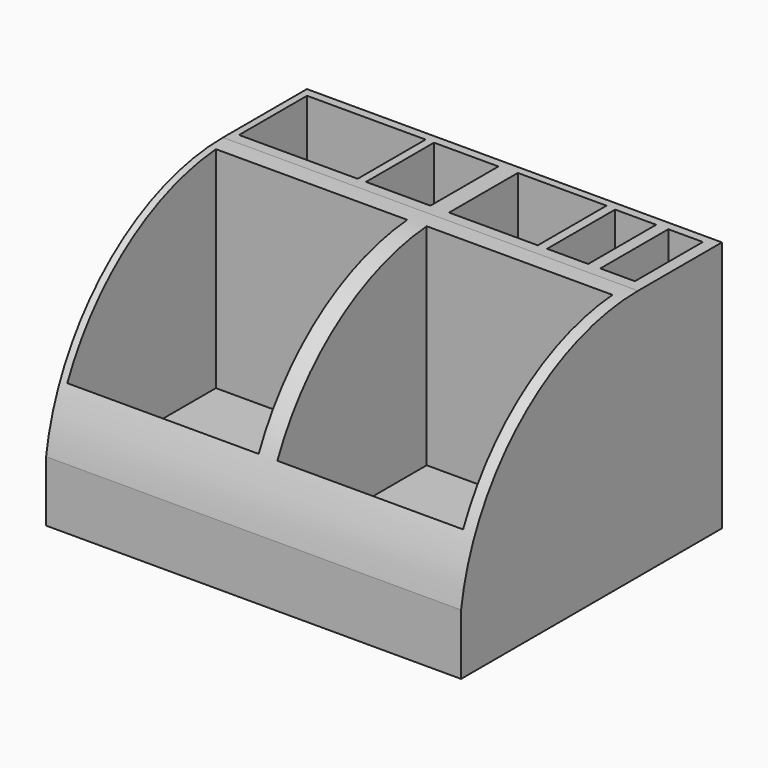
from build123d import *

# Parameters (mm, degrees)
F0_W        = 142.3350870609
F0_H        = 111.8143312633
F1_DEPTH    = 65.532
F2_T1_DEPTH = 521.5375533391
F4_DEPTH    = 20.828
F3_W        = 65.6352208462
F3_H        = 63.7141903862
F3_W_2      = 63.7141834013
F3_H_2      = 64.0343613923
F3_W_3      = 30.4163205437
F3_H_3      = 29.4558089226
F3_W_4      = 22.0918541308
F3_H_4      = 29.1356351227
F3_W_5      = 14.0875652432
F3_W_6      = 11.8463523686
F3_W_7      = 40.6618192792
F5_DEPTH    = 72.39


# Not quite as in the source:
# - a fillet or chamfer that OpenCascade refuses, or shapes differently, is made with other operations: its cross-section is extruded or revolved along the edge and cut away or added


with BuildPart() as f1:
    # F0 (on Top) → F1 (new body)
    with BuildSketch(Plane.XY):
        with Locations((-0.4278570414, 0.1426208764)):
            Rectangle(F0_W, F0_H)
    extrude(amount=F1_DEPTH)

    # F2: fillet of radius 76.6512806053 on 1 edges, made by hand

    # F2_s2 → F2_t1 (cut)
    with BuildSketch(Plane.YZ.offset(-261.1966337109)):
        with BuildLine():
            ThreePointArc((-55.7645447552, 0), (-30.0394768726, 46.8795379871), (20.0759485004, 65.532))
            Line((20.0759485004, 65.532), (-55.7645447552, 65.532))
            Line((-55.7645447552, 65.532), (-55.7645447552, 0))
        make_face()
    extrude(amount=F2_T1_DEPTH, mode=Mode.SUBTRACT)

    # F4 (add): a face of the model
    f4_faces = [f1.faces().sort_by_distance(p)[0] for p in [
        (-0.4278570414, 0.1426208764, 0),
    ]]
    extrude(f4_faces, amount=F4_DEPTH)

    # F3 (on face) → F5 (cut)
    with BuildSketch(Plane.XY.offset(65.532)):
        with Locations((-36.3275922136, -17.8819601424)):
            Rectangle(F3_W, F3_H)
        with Locations((34.7505474929, -17.7218746394)):
            Rectangle(F3_W_2, F3_H_2)
        with Locations((18.1016160641, 38.6283630505)):
            Rectangle(F3_W_3, F3_H_3)
        with Locations((-14.555908856, 38.4682761505)):
            Rectangle(F3_W_4, F3_H_4)
        with Locations((43.5552746058, 38.4682761505)):
            Rectangle(F3_W_5, F3_H_4)
        with Locations((60.6844630092, 38.4682761505)):
            Rectangle(F3_W_6, F3_H_4)
        with Locations((-48.8142929971, 38.4682761505)):
            Rectangle(F3_W_7, F3_H_4)
    extrude(amount=-F5_DEPTH, mode=Mode.SUBTRACT)


solid = f1.part
